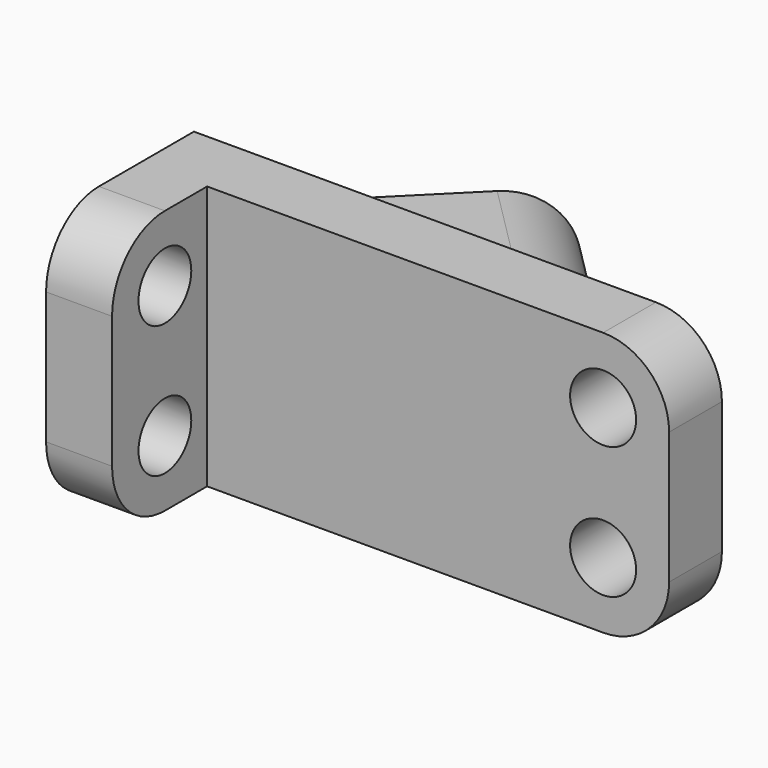
from build123d import *

# Parameters (mm, degrees)
F1_DEPTH  = 100
F2_R      = 25
F3_START  = 25
F3_DEPTH  = 50
F4_R      = 24.99999
F6_D      = 25
F6_DEPTH  = 195
F6_TIP    = 7.5107577378
F8_D      = 25
F8_DEPTH  = 195
F8_TIP    = 7.5107577378
F9_R      = 15
F10_DEPTH = 50


# Not quite as in the source:
# - a fillet or chamfer is up to 0.001 mm smaller than in the source, because OpenCascade refuses the exact size


with BuildPart() as f1:
    # F0 (on Top) → F1 (new body)
    with BuildSketch(Plane.XY):
        Polygon((0, 70), (0, 0), (25, 0), (25, 45), (200, 45), (200, 70), (163, 70), align=None)
    extrude(amount=F1_DEPTH)

    # F2
    f2_edges = [f1.edges().sort_by_distance(p)[0] for p in [
        (200, 57.5, 100),
        (200, 57.5, 0),
        (12.5, 0, 100),
        (12.5, 0, 0),
    ]]
    fillet(f2_edges, radius=F2_R)

    # F0 (on Top) → F3 (join)
    with BuildSketch(Plane.XY.offset(F3_START)):
        Polygon((17.6776695297, 87.6776695297), (0, 70), (163, 70), (81.5, 151.5), (28.2842712475, 98.2842712475), (38.8908729653, 87.6776695297), (28.2842712475, 77.0710678119), align=None)
    extrude(amount=F3_DEPTH)

    # F4 (radius 25 in the source; OpenCascade refuses exactly that, so slightly less here)
    f4_edges = [f1.edges().sort_by_distance(p)[0] for p in [
        (122.25, 110.75, 75),
        (122.25, 110.75, 25),
    ]]
    fillet(f4_edges, radius=F4_R)

    # F6
    with Locations(Plane(origin=(0, 70, 0), x_dir=(-1, 0, 0), z_dir=(0, 1, 0))):
        with Locations((-175, 25), (-175, 75)):
            Hole(F6_D / 2, depth=F6_DEPTH)
            with Locations((0, 0, -(F6_DEPTH + F6_TIP / 2))):  # 118° drill point
                Cone(0, F6_D / 2, F6_TIP, mode=Mode.SUBTRACT)

    # F8
    with Locations(Plane(origin=(0, 0, 0), x_dir=(0, -1, 0), z_dir=(-1, 0, 0))):
        with Locations((-25, 25), (-25, 75)):
            Hole(F8_D / 2, depth=F8_DEPTH)
            with Locations((0, 0, -(F8_DEPTH + F8_TIP / 2))):  # 118° drill point
                Cone(0, F8_D / 2, F8_TIP, mode=Mode.SUBTRACT)

    # F9 (on face) → F10 (cut)
    with BuildSketch(Plane(origin=(-35, 35, 0), x_dir=(-0.7071067812, -0.7071067812, 0), z_dir=(-0.7071067812, 0.7071067812, 0))):
        with Locations((-139.7558800165, 50)):
            Circle(F9_R)
    extrude(amount=-F10_DEPTH, mode=Mode.SUBTRACT)


solid = f1.part
